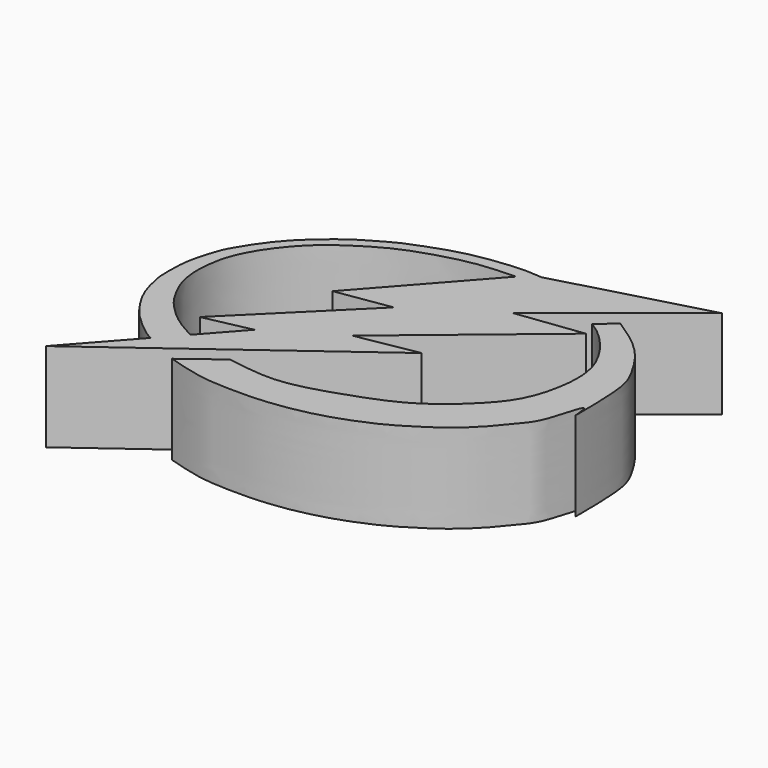
from build123d import *

# Parameters (mm, degrees)
F1_DEPTH = 10


# Not quite as in the source:
# - a feature of the source that left no trace in its solid (it failed there, or was rolled back) is left out


with BuildPart() as f1:
    # F0 (on Top) → F1 (new body)
    with BuildSketch(Plane.XY):
        with BuildLine():
            Line((6.7712266664, -34.9485791715), (0.5917352391, -41.8838895857))
            Line((0.5917352391, -41.8838895857), (27.1167848259, -22.357461974))
            Line((27.1167848259, -22.357461974), (20.3185230494, -23.5622171313))
            Line((20.3185230494, -23.5622171313), (36.0663942993, -10.4820188135))
            Line((36.0663942993, -10.4820188135), (28.5797007382, -11.4286132157))
            Line((28.5797007382, -11.4286132157), (42.9507084191, 0))
            Line((42.9507084191, 0), (26.3422988355, -4.5442981645))
            add(Edge.make_bspline(
                [(26.3422988355, -4.5442981645), (25.8078429871, -4.4981026613), (24.6477537147, -4.397830753), (22.4411040837, -4.4962992569), (18.9409738337, -5.0124200177), (16.7713353432, -5.6015179544), (14.6053514546, -6.3950040748), (12.3677600296, -7.2325630823), (10.5945935269, -8.3377494254), (9.1178266686, -9.1299999948), (7.6881476544, -10.1960688332), (6.5697003284, -11.1406239757), (4.9996008275, -12.5466240058), (3.750420964, -13.9955143391), (2.6532822105, -15.5087208498), (2.2179365417, -16.2518261338), (1.3648002526, -17.6273689957), (0.9772244672, -18.6865585645), (0.3437092481, -20.6764003422), (0.132981441, -22.1072539999), (0.0913115279, -23.1519385454), (0.0489551854, -25.0797474167), (0.2610416036, -26.281731387), (0.8041219133, -28.4012577684), (1.7025670054, -30.0294676037), (2.616107057, -31.396802322), (3.7462102067, -32.7044331363), (5.7805997809, -34.4198344322), (6.4926618956, -34.799895889), (6.7712266664, -34.9485791715)],
                knots=[0, 0, 0, 0, 0.0353278959, 0.0766826917, 0.1285695112, 0.1703473888, 0.2118270215, 0.2546772453, 0.2943867249, 0.3302100033, 0.3665306376, 0.4001694433, 0.4398383629, 0.479021361, 0.5158887562, 0.5420789353, 0.5761228769, 0.606393396, 0.6460584058, 0.6791288299, 0.7075532301, 0.7451233272, 0.7764294046, 0.8166786602, 0.85474218, 0.8893888486, 0.9263626494, 0.9711924406, 1, 1, 1, 1], degree=3))
        make_face()
        with BuildLine():
            add(Edge.make_bspline(
                [(9.1226673937, -32.3095316776), (8.7587950877, -32.1266297091), (7.9109419803, -31.6643872593), (6.3065914642, -30.6564466653), (4.3755403597, -28.8233696959), (3.3989004542, -27.3881165551), (2.5758203214, -25.7477529854), (2.2085789347, -24.6529328483), (1.8890714, -22.9599893607), (1.9732711776, -21.3249194942), (2.2644433552, -19.0924237867), (3.3274707055, -16.7010730558), (4.740620184, -14.6129601331), (7.0909150889, -11.841048354), (11.2680390158, -9.1230428498), (13.9872648451, -7.8363900411), (17.3522243585, -6.7497538917), (20.6235545311, -5.9954361088), (23.2015225837, -5.8897433856), (24.5341658592, -5.835107062)],
                knots=[0, 0, 0, 0, 0.0429794677, 0.0950219776, 0.1558685653, 0.2060635337, 0.2556475504, 0.2962629889, 0.3443857243, 0.3925423903, 0.4483863982, 0.5085603685, 0.5674950025, 0.6390537502, 0.7223159975, 0.7879276623, 0.8571201686, 0.9259668406, 1, 1, 1, 1], degree=3))
            Line((24.5341658592, -5.835107062), (13.6879626662, -18.0547665805))
            Line((13.6879626662, -18.0547665805), (19.7997130454, -17.1081721783))
            Line((19.7997130454, -17.1081721783), (7.6622935012, -29.1557237506))
            Line((7.6622935012, -29.1557237506), (12.9184202345, -28.0495169957))
            Line((12.9184202345, -28.0495169957), (9.1226673937, -32.3095316776))
        make_face(mode=Mode.SUBTRACT)
    extrude(amount=F1_DEPTH)


with BuildPart() as f1b:
    # F0 (on Top) → F1, piece 2 (new body)
    with BuildSketch(Plane.XY):
        with BuildLine():
            Line((37.2131988406, -7.0866299793), (35.3583954275, -8.7139569223))
            add(Edge.make_bspline(
                [(35.3583954275, -8.7139569223), (36.3378810059, -9.2990359155), (38.1208264676, -10.7906681601), (41.0136616979, -15.0142954637), (40.7302854757, -19.9797435506), (39.4496938965, -24.0629309921), (36.322337101, -27.4297919783), (32.782132289, -30.2563763173), (29.2132154423, -31.8871735641), (24.4225596815, -33.5433536559), (19.9292022469, -34.651918561), (16.4291285285, -34.0651901088), (14.7506631911, -33.8126718998)],
                knots=[0, 0, 0, 0, 0.0873677066, 0.1916575682, 0.2952562075, 0.3918638462, 0.4921691286, 0.5920103036, 0.6855182634, 0.7911290325, 0.8928070809, 1, 1, 1, 1], degree=3))
            Line((14.7506631911, -33.8126718998), (10.7073178515, -36.8629135191))
            add(Edge.make_bspline(
                [(37.2131988406, -7.0866299793), (38.0039627841, -7.5995621332), (39.5111572818, -8.5752585824), (40.9685114935, -9.8676683125), (42.2534586977, -11.1790878844), (44.0407365865, -14.0321723947), (44.939816218, -16.2946280399), (45.0361378773, -20.6451806436), (45.0791530187, -24.2478358004), (44.8550437466, -19.8645032564), (43.5647115361, -25.9124618391), (42.0142819502, -27.4477535289), (40.3086929783, -29.765417743), (37.5751807702, -32.2458055729), (35.21921375, -33.6717801447), (33.204261961, -35.0104294821), (28.1544510173, -37.1538405557), (22.4083374627, -38.2224659701), (17.8732038248, -38.2071837918), (14.6349893051, -38.0309131912), (12.0295608101, -37.2561196962), (10.7073178515, -36.8629135191)],
                knots=[0, 0, 0, 0, 0.0494275049, 0.0902093733, 0.1305463147, 0.1840414273, 0.2308698687, 0.2966276603, 0.3375458303, 0.374157977, 0.4329395539, 0.48168968, 0.5306598249, 0.5880880085, 0.6367450558, 0.6823000992, 0.7512595946, 0.8244265897, 0.8869536012, 0.9401063655, 1, 1, 1, 1], degree=3))
        make_face()
    extrude(amount=F1_DEPTH)


solid = Compound([f1.part, f1b.part])
